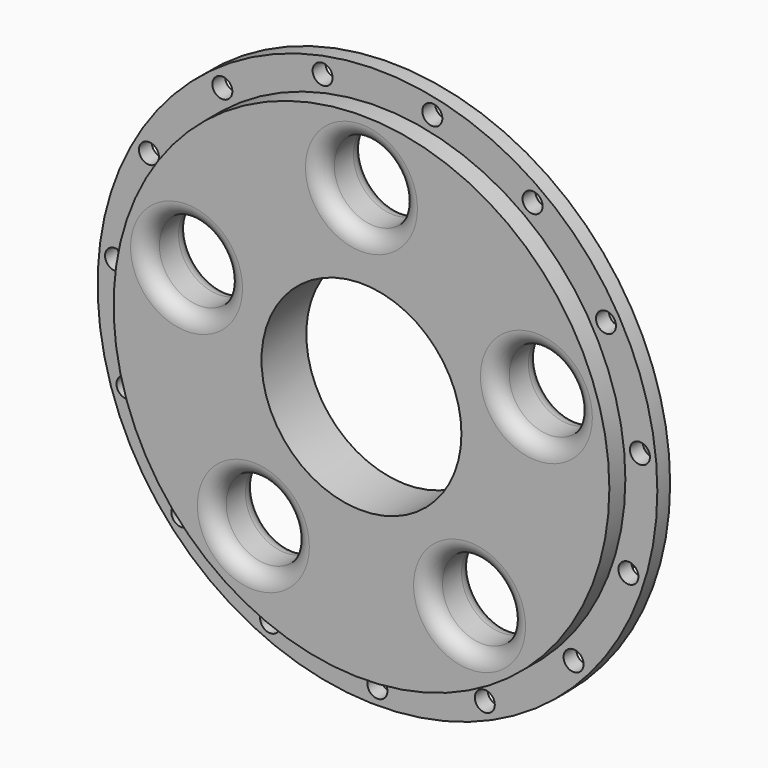
from build123d import *

# Parameters (mm, degrees)
F0_R          = 35
F1_DEPTH      = 3
F1_DEPTH_BACK = 4
F2_R          = 12.5
F3_DEPTH      = 25
F4_R          = 5
F5_DEPTH      = 25
F7_R          = 2
F8_R          = 35.2185904309
F8_R_2        = 31
F9_DEPTH      = 2.5
F10_R         = 40.9097985185
F10_R_2       = 31
F11_DEPTH     = 2.5
F12_R         = 1.25
F13_DEPTH     = 25


# Not quite as in the source:
# - a feature names something its author has since deleted; it is built from what else it names


with BuildPart() as f1:
    # F0 (on Front) → F1 (new body, two sides)
    with BuildSketch(Plane.XZ) as f1_sk:
        Circle(F0_R)
    extrude(amount=-F1_DEPTH)
    extrude(f1_sk.sketch, amount=F1_DEPTH_BACK)

    # F2 (on face) → F3 (cut)
    with BuildSketch(Plane.XZ.offset(4)):
        Circle(F2_R)
    extrude(amount=-F3_DEPTH, mode=Mode.SUBTRACT)

    # F4 (on face) → F5 (cut)
    with BuildSketch(Plane.XZ.offset(4)):
        with Locations((0, 23)):
            Circle(F4_R)
        with Locations((-21.8742998748, 7.1073908706)):
            Circle(F4_R)
        with Locations((-13.5190608027, -18.6073908706)):
            Circle(F4_R)
        with Locations((13.5190608027, -18.6073908706)):
            Circle(F4_R)
        with Locations((21.8742998748, 7.1073908706)):
            Circle(F4_R)
    extrude(amount=-F5_DEPTH, mode=Mode.SUBTRACT)

    # F7
    f7_edges = [f1.edges().sort_by_distance(p)[0] for p in [
        (-5, -4, 23),
        (-26.8743, -4, 7.107391),
        (-18.519061, -4, -18.607391),
        (-26.8743, 3, 7.107391),
        (-18.519061, 3, -18.607391),
        (-5, 3, 23),
        (8.519061, -4, -18.607391),
        (8.519061, 3, -18.607391),
        (16.8743, -4, 7.107391),
        (16.8743, 3, 7.107391),
    ]]
    fillet(f7_edges, radius=F7_R)

    # F8 (on face) → F9 (cut)
    with BuildSketch(Plane.XZ.offset(4)):
        Circle(F8_R)
        Circle(F8_R_2, mode=Mode.SUBTRACT)
    extrude(amount=-F9_DEPTH, mode=Mode.SUBTRACT)

    # F10 (on face) → F11 (cut)
    with BuildSketch(Plane(origin=(0, 3, 0), x_dir=(-1, 0, 0), z_dir=(0, 1, 0))):
        Circle(F10_R)
        Circle(F10_R_2, mode=Mode.SUBTRACT)
    extrude(amount=-F11_DEPTH, mode=Mode.SUBTRACT)

    # F12 (on face) → F13 (cut)
    with BuildSketch(Plane.XZ.offset(1.5)):
        with Locations((6.861085797, 32.2788708242)):
            Circle(F12_R)
        with Locations((-6.861085797, 32.2788708242)):
            Circle(F12_R)
        with Locations((-19.3969133257, 26.6975608144)):
            Circle(F12_R)
        with Locations((-28.5788383249, 16.5)):
            Circle(F12_R)
        with Locations((-32.8192225472, 3.4494392878)):
            Circle(F12_R)
        with Locations((-31.3848650377, -10.1975608144)):
            Circle(F12_R)
        with Locations((-24.5237792408, -22.0813100098)):
            Circle(F12_R)
        with Locations((-13.4223092215, -30.1470001022)):
            Circle(F12_R)
        with Locations((0, -33)):
            Circle(F12_R)
        with Locations((13.4223092215, -30.1470001022)):
            Circle(F12_R)
        with Locations((24.5237792408, -22.0813100098)):
            Circle(F12_R)
        with Locations((31.3848650377, -10.1975608144)):
            Circle(F12_R)
        with Locations((32.8192225472, 3.4494392878)):
            Circle(F12_R)
        with Locations((28.5788383249, 16.5)):
            Circle(F12_R)
        with Locations((19.3969133257, 26.6975608144)):
            Circle(F12_R)
    extrude(amount=-F13_DEPTH, mode=Mode.SUBTRACT)


solid = f1.part
